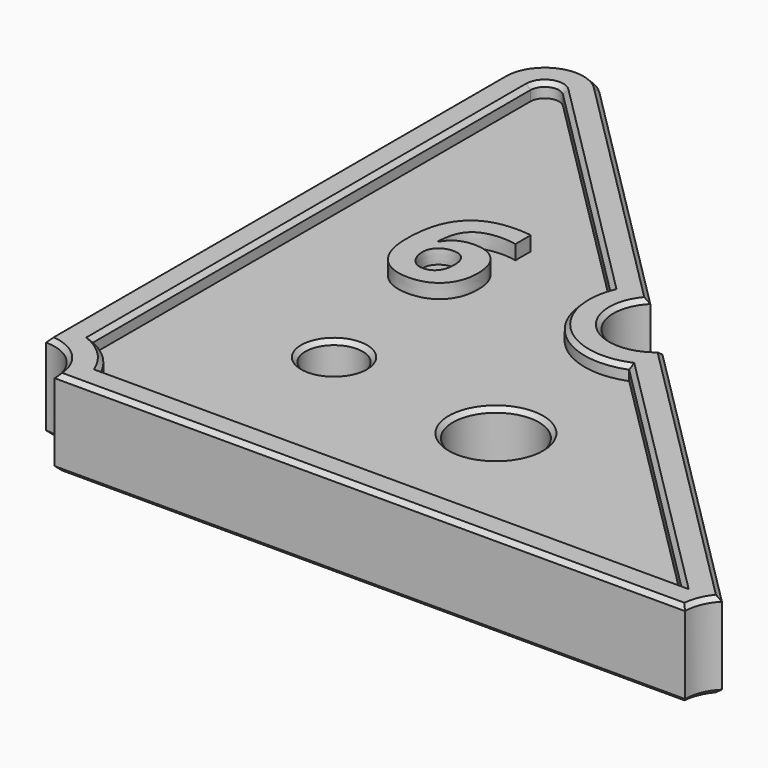
from build123d import *

# Parameters (mm, degrees)
F0_R         = 2
F0_R_2       = 3
F0_TEXT_SIZE = 11.1111111111
F1_DEPTH     = 5
F3_DEPTH     = 1
F4_SIZE      = 0.3


# Not quite as in the source:
# - Text() gives the source's letters only with a copy of the font that has no kerning and outlines rounded to 1/6400 em; it was checked with that copy


with BuildPart() as f1:
    # F0 (on Top) → F1 (new body)
    with BuildSketch(Plane.XY):
        with BuildLine():
            ThreePointArc((-19.8786796564, 19.8786796564), (-23.1480502971, 20.5289979104), (-25, 17.7573593129))
            Line((-25, 17.7573593129), (-25, -22))
            ThreePointArc((-25, -22), (-22.8786796564, -22.8786796564), (-22, -25))
            Line((-22, -25), (22, -25))
            ThreePointArc((22, -25), (22.2283614025, -23.8519497029), (22.8786796564, -22.8786796564))
            Line((22.8786796564, -22.8786796564), (2.1213203436, -2.1213203436))
            ThreePointArc((2.1213203436, -2.1213203436), (-2.1213203436, -2.1213203436), (-2.1213203436, 2.1213203436))
            Line((-2.1213203436, 2.1213203436), (-19.8786796564, 19.8786796564))
        make_face()
        with Locations((-12.5, -12.5)):
            Circle(F0_R, mode=Mode.SUBTRACT)
        with Locations((0, -14)):
            Circle(F0_R_2, mode=Mode.SUBTRACT)
        with BuildLine():
            add(Edge.make_bspline(
                [(-16.609375, -2.5138888889), (-16.9644097222, -1.7326388889), (-16.9644097222, -0.6302083333)],
                knots=[0, 0, 0, 1, 1, 1], degree=2))
            add(Edge.make_bspline(
                [(-16.9644097222, -0.6302083333), (-16.9644097222, 1.7239583333), (-15.96875, 2.8741319444)],
                knots=[0, 0, 0, 1, 1, 1], degree=2))
            add(Edge.make_bspline(
                [(-15.96875, 2.8741319444), (-14.9730902778, 4.0243055556), (-12.9869791667, 4.0243055556)],
                knots=[0, 0, 0, 1, 1, 1], degree=2))
            add(Edge.make_bspline(
                [(-12.9869791667, 4.0243055556), (-12.3098958333, 4.0243055556), (-11.9244791667, 3.9427083333)],
                knots=[0, 0, 0, 1, 1, 1], degree=2))
            Line((-11.9244791667, 3.9427083333), (-11.9244791667, 2.6024305556))
            add(Edge.make_bspline(
                [(-11.9244791667, 2.6024305556), (-12.4071180556, 2.7118055556), (-12.8793402778, 2.7118055556)],
                knots=[0, 0, 0, 1, 1, 1], degree=2))
            add(Edge.make_bspline(
                [(-12.8793402778, 2.7118055556), (-13.7421875, 2.7118055556), (-14.2873263889, 2.4513888889)],
                knots=[0, 0, 0, 1, 1, 1], degree=2))
            add(Edge.make_bspline(
                [(-14.2873263889, 2.4513888889), (-14.8324652778, 2.1909722222), (-15.1032986111, 1.6805555556)],
                knots=[0, 0, 0, 1, 1, 1], degree=2))
            add(Edge.make_bspline(
                [(-15.1032986111, 1.6805555556), (-15.3741319444, 1.1701388889), (-15.4227430556, 0.2326388889)],
                knots=[0, 0, 0, 1, 1, 1], degree=2))
            Line((-15.4227430556, 0.2326388889), (-15.3532986111, 0.2326388889))
            add(Edge.make_bspline(
                [(-15.3532986111, 0.2326388889), (-14.8151041667, 1.1545138889), (-13.6328125, 1.1545138889)],
                knots=[0, 0, 0, 1, 1, 1], degree=2))
            add(Edge.make_bspline(
                [(-13.6328125, 1.1545138889), (-12.5703125, 1.1545138889), (-11.9678819444, 0.4869791667)],
                knots=[0, 0, 0, 1, 1, 1], degree=2))
            add(Edge.make_bspline(
                [(-11.9678819444, 0.4869791667), (-11.3654513889, -0.1805555556), (-11.3654513889, -1.3576388889)],
                knots=[0, 0, 0, 1, 1, 1], degree=2))
            add(Edge.make_bspline(
                [(-11.3654513889, -1.3576388889), (-11.3654513889, -2.6267361111), (-12.0815972222, -3.3680555556)],
                knots=[0, 0, 0, 1, 1, 1], degree=2))
            add(Edge.make_bspline(
                [(-12.0815972222, -3.3680555556), (-12.7977430556, -4.109375), (-14.0668402778, -4.109375)],
                knots=[0, 0, 0, 1, 1, 1], degree=2))
            add(Edge.make_bspline(
                [(-14.0668402778, -4.109375), (-14.9453125, -4.109375), (-15.5998263889, -3.7022569444)],
                knots=[0, 0, 0, 1, 1, 1], degree=2))
            add(Edge.make_bspline(
                [(-15.5998263889, -3.7022569444), (-16.2543402778, -3.2951388889), (-16.609375, -2.5138888889)],
                knots=[0, 0, 0, 1, 1, 1], degree=2))
        make_face(mode=Mode.SUBTRACT)
        with Locations((-17.3550347222, -4)):
            Text('6', F0_TEXT_SIZE, font='Open Sans', font_style=FontStyle.BOLD, text_align=(TextAlign.LEFT, TextAlign.BOTTOM))
        with BuildLine():
            add(Edge.make_bspline(
                [(-14.9600694444, -2.3237847222), (-14.6206597222, -2.7690972222), (-14.0998263889, -2.7690972222)],
                knots=[0, 0, 0, 1, 1, 1], degree=2))
            add(Edge.make_bspline(
                [(-14.0998263889, -2.7690972222), (-13.5633680556, -2.7690972222), (-13.2751736111, -2.4079861111)],
                knots=[0, 0, 0, 1, 1, 1], degree=2))
            add(Edge.make_bspline(
                [(-13.2751736111, -2.4079861111), (-12.9869791667, -2.046875), (-12.9869791667, -1.3802083333)],
                knots=[0, 0, 0, 1, 1, 1], degree=2))
            add(Edge.make_bspline(
                [(-12.9869791667, -1.3802083333), (-12.9869791667, -0.7986111111), (-13.2560763889, -0.4652777778)],
                knots=[0, 0, 0, 1, 1, 1], degree=2))
            add(Edge.make_bspline(
                [(-13.2560763889, -0.4652777778), (-13.5251736111, -0.1319444444), (-14.0668402778, -0.1319444444)],
                knots=[0, 0, 0, 1, 1, 1], degree=2))
            add(Edge.make_bspline(
                [(-14.0668402778, -0.1319444444), (-14.5772569444, -0.1319444444), (-14.9383680556, -0.4626736111)],
                knots=[0, 0, 0, 1, 1, 1], degree=2))
            add(Edge.make_bspline(
                [(-14.9383680556, -0.4626736111), (-15.2994791667, -0.7934027778), (-15.2994791667, -1.2326388889)],
                knots=[0, 0, 0, 1, 1, 1], degree=2))
            add(Edge.make_bspline(
                [(-15.2994791667, -1.2326388889), (-15.2994791667, -1.8784722222), (-14.9600694444, -2.3237847222)],
                knots=[0, 0, 0, 1, 1, 1], degree=2))
        make_face()
    extrude(amount=-F1_DEPTH)

    # F0 (on Top) + F2 (on face) → F3 (join)
    with BuildSketch(Plane.XY):
        with Locations((-17.3550347222, -4)):
            Text('6', F0_TEXT_SIZE, font='Open Sans', font_style=FontStyle.BOLD, text_align=(TextAlign.LEFT, TextAlign.BOTTOM))
    with BuildSketch(Plane.XY):
        with BuildLine():
            ThreePointArc((2.1213203436, -2.1213203436), (-2.1213203436, -2.1213203436), (-2.1213203436, 2.1213203436))
            Line((-2.1213203436, 2.1213203436), (-19.8786796564, 19.8786796564))
            ThreePointArc((-19.8786796564, 19.8786796564), (-23.1480502971, 20.5289979104), (-25, 17.7573593129))
            Line((-25, 17.7573593129), (-25, -22))
            ThreePointArc((-25, -22), (-22.8786796564, -22.8786796564), (-22, -25))
            Line((-22, -25), (22, -25))
            ThreePointArc((22, -25), (22.2283614025, -23.8519497029), (22.8786796564, -22.8786796564))
            Line((22.8786796564, -22.8786796564), (2.1213203436, -2.1213203436))
        make_face()
        with BuildLine():
            Line((1.8261567868, -4.6545839116), (20.1715728753, -23))
            Line((20.1715728753, -23), (-20.417424305, -23))
            ThreePointArc((-20.417424305, -23), (-21.4644660941, -21.4644660941), (-23, -20.417424305))
            Line((-23, -20.417424305), (-23, 17.7573593129))
            ThreePointArc((-23, 17.7573593129), (-22.3826834324, 18.6812388454), (-21.2928932188, 18.4644660941))
            Line((-21.2928932188, 18.4644660941), (-4.6545839116, 1.8261567868))
            ThreePointArc((-4.6545839116, 1.8261567868), (-3.5355339059, -3.5355339059), (1.8261567868, -4.6545839116))
        make_face(mode=Mode.SUBTRACT)
    extrude(amount=F3_DEPTH)

    # F4
    f4_edges = [f1.edges().sort_by_distance(p)[0] for p in [
        (12.5, -12.5, 1),
        (-2.12132, -2.12132, 1),
        (-11, 11, 1),
        (-23.14805, 20.528998, 1),
        (-25, -2.12132, 1),
        (-22.87868, -22.87868, 1),
        (0, -25, 1),
        (22.228361, -23.85195, 1),
        (-22.382683, 18.681239, 1),
        (-12.973739, 10.145311, 1),
        (-3.535534, -3.535534, 1),
        (10.998865, -13.827292, 1),
        (-0.122926, -23, 1),
        (-21.464466, -21.464466, 1),
        (-23, -1.330032, 1),
        (-14.5, -12.5, 0),
        (-3, -14, 0),
        (-11, 11, -5),
        (-23.14805, 20.528998, -5),
        (-25, -2.12132, -5),
        (-22.87868, -22.87868, -5),
        (0, -25, -5),
        (22.228361, -23.85195, -5),
        (12.5, -12.5, -5),
        (-2.12132, -2.12132, -5),
        (-14.5, -12.5, -5),
        (-3, -14, -5),
    ]]
    chamfer(f4_edges, length=F4_SIZE)


solid = f1.part
